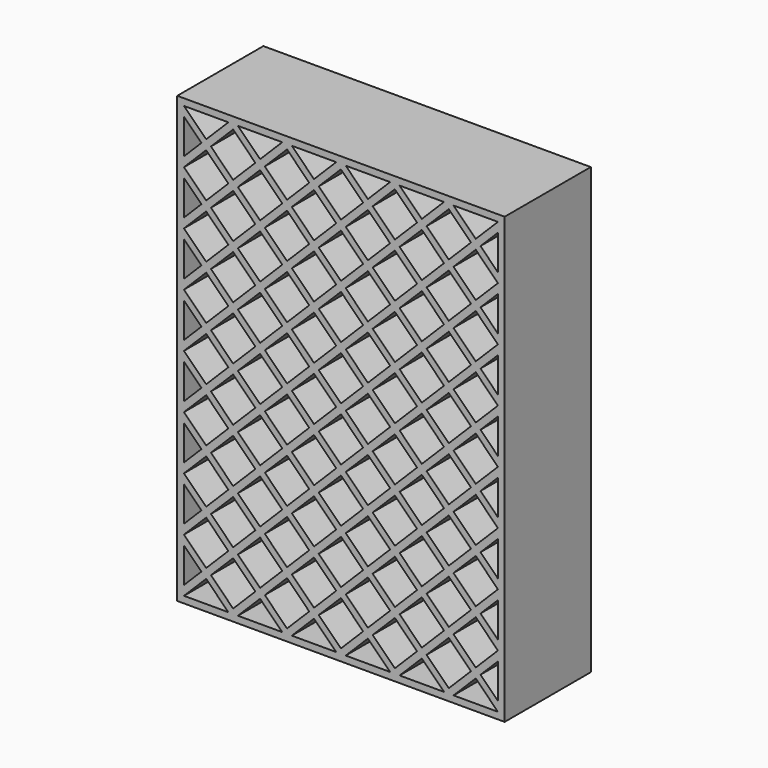
from build123d import *

# Parameters (mm, degrees)
F0_W     = 927.1
F0_H     = 1259.3694764796
F1_DEPTH = 152.4


with BuildPart() as f1:
    # F0 (on Front) → F1 (new body, symmetric)
    with BuildSketch(Plane.XZ):
        with Locations((444.5, 610.6347382398)):
            Rectangle(F0_W, F0_H)
        Polygon((125.6782297091, 0), (0, 0), (0, 26.9407683632), (0, 125.6782297091), (0, 152.6189980723), (0, 152.6643540582), (0, 179.6051224214), (0, 278.3425837673), (0, 305.2833521305), (0, 305.3287081164), (0, 332.2694764796), (0, 431.0069378255), (0, 457.9477061887), (0, 457.9930621745), (0, 484.9338305377), (0, 583.6712918836), (0, 610.6120602469), (0, 610.6574162327), (0, 637.5981845959), (0, 736.3356459418), (0, 763.276414305), (0, 763.3217702909), (0, 790.2625386541), (0, 889), (0, 915.9407683632), (0, 915.9861243491), (0, 942.9268927123), (0, 1041.6643540582), (0, 1068.6051224214), (0, 1068.6504784072), (0, 1095.5912467704), (0, 1194.3287081164), (0, 1221.2694764796), (125.6782297091, 1221.2694764796), (125.700907702, 1221.2921544725), (125.723585695, 1221.2694764796), (152.6189980723, 1221.2694764796), (152.6416760653, 1221.2921544725), (152.6643540582, 1221.2694764796), (278.3425837673, 1221.2694764796), (278.3652617602, 1221.2921544725), (278.3879397531, 1221.2694764796), (305.2833521305, 1221.2694764796), (305.3060301234, 1221.2921544725), (305.3287081164, 1221.2694764796), (431.0069378255, 1221.2694764796), (431.0296158184, 1221.2921544725), (431.0522938113, 1221.2694764796), (457.9477061887, 1221.2694764796), (457.9703841816, 1221.2921544725), (457.9930621745, 1221.2694764796), (583.6712918836, 1221.2694764796), (583.6939698766, 1221.2921544725), (583.7166478695, 1221.2694764796), (610.6120602469, 1221.2694764796), (610.6347382398, 1221.2921544725), (610.6574162327, 1221.2694764796), (736.3356459418, 1221.2694764796), (736.3583239347, 1221.2921544725), (736.3810019277, 1221.2694764796), (763.276414305, 1221.2694764796), (763.299092298, 1221.2921544725), (763.3217702909, 1221.2694764796), (889, 1221.2694764796), (889, 1194.3287081164), (889, 1095.5912467704), (889, 1068.6504784072), (889, 1068.6051224214), (889, 1041.6643540582), (889, 942.9268927123), (889, 915.9861243491), (889, 915.9407683632), (889, 889), (889, 790.2625386541), (889, 763.3217702909), (889, 763.276414305), (889, 736.3356459418), (889, 637.5981845959), (889, 610.6574162327), (889, 610.6120602469), (889, 583.6712918836), (889, 484.9338305377), (889, 457.9930621745), (889, 457.9477061887), (889, 431.0069378255), (889, 332.2694764796), (889, 305.3287081164), (889, 305.2833521305), (889, 278.3425837673), (889, 179.6051224214), (889, 152.6643540582), (889, 152.6189980723), (889, 125.6782297091), (889, 26.9407683632), (889, 0), (763.3217702909, 0), (763.276414305, 0), (736.3810019277, 0), (736.3356459418, 0), (610.6574162327, 0), (610.6120602469, 0), (583.7166478695, 0), (583.6712918836, 0), (457.9930621745, 0), (457.9477061887, 0), (431.0522938113, 0), (431.0069378255, 0), (305.3287081164, 0), (305.2833521305, 0), (278.3879397531, 0), (278.3425837673, 0), (152.6643540582, 0), (152.6189980723, 0), (125.723585695, 0), align=None, mode=Mode.SUBTRACT)
        Polygon((125.700907702, 915.9634463561), (139.1712918836, 902.4930621745), (152.6416760653, 915.9634463561), (139.1712918836, 929.4338305377), align=None)
        Polygon((125.700907702, 1068.6278004143), (139.1712918836, 1055.1574162327), (152.6416760653, 1068.6278004143), (139.1712918836, 1082.0981845959), align=None)
        Polygon((291.8356459418, 1082.0981845959), (305.3060301234, 1068.6278004143), (368.1678229709, 1131.4895932618), (354.6974387893, 1144.9599774434), align=None)
        Polygon((125.700907702, 763.299092298), (139.1712918836, 749.8287081164), (152.6416760653, 763.299092298), (139.1712918836, 776.7694764796), align=None)
        Polygon((291.8356459418, 776.7694764796), (305.3060301234, 763.299092298), (368.1678229709, 826.1608851454), (354.6974387893, 839.631269327), align=None)
        Polygon((291.8356459418, 902.4930621745), (354.6974387893, 839.631269327), (368.1678229709, 853.1016535086), (305.3060301234, 915.9634463561), align=None)
        Polygon((354.6974387893, 992.2956233852), (368.1678229709, 978.8252392036), (381.6382071525, 992.2956233852), (368.1678229709, 1005.7660075668), align=None)
        Polygon((62.8391148546, 853.1016535086), (76.3094990362, 839.631269327), (139.1712918836, 902.4930621745), (125.700907702, 915.9634463561), align=None)
        Polygon((49.368730673, 1144.9599774434), (62.8391148546, 1131.4895932618), (76.3094990362, 1144.9599774434), (62.8391148546, 1158.430361625), align=None)
        Polygon((215.5034689127, 978.8252392036), (278.3652617602, 915.9634463561), (291.8356459418, 929.4338305377), (228.9738530943, 992.2956233852), align=None)
        Polygon((278.3652617602, 1068.6278004143), (291.8356459418, 1055.1574162327), (305.3060301234, 1068.6278004143), (291.8356459418, 1082.0981845959), align=None)
        Polygon((62.8391148546, 826.1608851454), (125.700907702, 763.299092298), (139.1712918836, 776.7694764796), (76.3094990362, 839.631269327), align=None)
        Polygon((49.368730673, 992.2956233852), (62.8391148546, 978.8252392036), (76.3094990362, 992.2956233852), (62.8391148546, 1005.7660075668), align=None)
        Polygon((215.5034689127, 826.1608851454), (278.3652617602, 763.299092298), (291.8356459418, 776.7694764796), (228.9738530943, 839.631269327), align=None)
        Polygon((278.3652617602, 915.9634463561), (291.8356459418, 902.4930621745), (305.3060301234, 915.9634463561), (291.8356459418, 929.4338305377), align=None)
        Polygon((354.6974387893, 1144.9599774434), (368.1678229709, 1131.4895932618), (381.6382071525, 1144.9599774434), (368.1678229709, 1158.430361625), align=None)
        Polygon((139.1712918836, 902.4930621745), (202.0330847311, 839.631269327), (215.5034689127, 853.1016535086), (152.6416760653, 915.9634463561), align=None)
        Polygon((62.8391148546, 978.8252392036), (125.700907702, 915.9634463561), (139.1712918836, 929.4338305377), (76.3094990362, 992.2956233852), align=None)
        Polygon((215.5034689127, 1005.7660075668), (228.9738530943, 992.2956233852), (291.8356459418, 1055.1574162327), (278.3652617602, 1068.6278004143), align=None)
        Polygon((215.5034689127, 853.1016535086), (228.9738530943, 839.631269327), (291.8356459418, 902.4930621745), (278.3652617602, 915.9634463561), align=None)
        Polygon((278.3652617602, 763.299092298), (291.8356459418, 749.8287081164), (305.3060301234, 763.299092298), (291.8356459418, 776.7694764796), align=None)
        Polygon((291.8356459418, 929.4338305377), (305.3060301234, 915.9634463561), (368.1678229709, 978.8252392036), (354.6974387893, 992.2956233852), align=None)
        Polygon((49.368730673, 839.631269327), (62.8391148546, 826.1608851454), (76.3094990362, 839.631269327), (62.8391148546, 853.1016535086), align=None)
        Polygon((62.8391148546, 1005.7660075668), (76.3094990362, 992.2956233852), (139.1712918836, 1055.1574162327), (125.700907702, 1068.6278004143), align=None)
        Polygon((62.8391148546, 1131.4895932618), (125.700907702, 1068.6278004143), (139.1712918836, 1082.0981845959), (76.3094990362, 1144.9599774434), align=None)
        Polygon((202.0330847311, 992.2956233852), (215.5034689127, 978.8252392036), (228.9738530943, 992.2956233852), (215.5034689127, 1005.7660075668), align=None)
        Polygon((202.0330847311, 839.631269327), (215.5034689127, 826.1608851454), (228.9738530943, 839.631269327), (215.5034689127, 853.1016535086), align=None)
        Polygon((202.0330847311, 1144.9599774434), (215.5034689127, 1131.4895932618), (228.9738530943, 1144.9599774434), (215.5034689127, 1158.430361625), align=None)
        Polygon((139.1712918836, 929.4338305377), (152.6416760653, 915.9634463561), (215.5034689127, 978.8252392036), (202.0330847311, 992.2956233852), align=None)
        Polygon((139.1712918836, 1055.1574162327), (202.0330847311, 992.2956233852), (215.5034689127, 1005.7660075668), (152.6416760653, 1068.6278004143), align=None)
        Polygon((139.1712918836, 1082.0981845959), (152.6416760653, 1068.6278004143), (215.5034689127, 1131.4895932618), (202.0330847311, 1144.9599774434), align=None)
        Polygon((354.6974387893, 839.631269327), (368.1678229709, 826.1608851454), (381.6382071525, 839.631269327), (368.1678229709, 853.1016535086), align=None)
        Polygon((215.5034689127, 1131.4895932618), (278.3652617602, 1068.6278004143), (291.8356459418, 1082.0981845959), (228.9738530943, 1144.9599774434), align=None)
        Polygon((291.8356459418, 1055.1574162327), (354.6974387893, 992.2956233852), (368.1678229709, 1005.7660075668), (305.3060301234, 1068.6278004143), align=None)
        Polygon((139.1712918836, 776.7694764796), (152.6416760653, 763.299092298), (215.5034689127, 826.1608851454), (202.0330847311, 839.631269327), align=None)
        Polygon((139.1712918836, 444.5), (202.0330847311, 381.6382071525), (215.5034689127, 395.1085913341), (152.6416760653, 457.9703841816), align=None)
        Polygon((431.0296158184, 152.6416760653), (368.1678229709, 89.7798832178), (381.6382071525, 76.3094990362), (444.5, 139.1712918836), align=None)
        Polygon((749.8287081164, 1055.1574162327), (812.6905009638, 992.2956233852), (826.1608851454, 1005.7660075668), (763.299092298, 1068.6278004143), align=None)
        Polygon((597.1643540582, 929.4338305377), (610.6347382398, 915.9634463561), (673.4965310873, 978.8252392036), (660.0261469057, 992.2956233852), align=None)
        Polygon((444.5, 902.4930621745), (507.3617928475, 839.631269327), (520.8321770291, 853.1016535086), (457.9703841816, 915.9634463561), align=None)
        Polygon((610.6347382398, 152.6416760653), (597.1643540582, 139.1712918836), (660.0261469057, 76.3094990362), (673.4965310873, 89.7798832178), align=None)
        Polygon((291.8356459418, 13.4477061887), (305.2833521305, 0), (305.3287081164, 0), (368.1678229709, 62.8391148546), (354.6974387893, 76.3094990362), align=None)
        Polygon((368.1678229709, 395.1085913341), (381.6382071525, 381.6382071525), (444.5, 444.5), (431.0296158184, 457.9703841816), align=None)
        Polygon((583.6939698766, 305.3060301234), (520.8321770291, 242.4442372759), (534.3025612107, 228.9738530943), (597.1643540582, 291.8356459418), align=None)
        Polygon((673.4965310873, 700.4372994505), (686.9669152689, 686.9669152689), (749.8287081164, 749.8287081164), (736.3583239347, 763.299092298), align=None)
        Polygon((444.5, 597.1643540582), (507.3617928475, 534.3025612107), (520.8321770291, 547.7729453923), (457.9703841816, 610.6347382398), align=None)
        Polygon((291.8356459418, 471.4407683632), (305.3060301234, 457.9703841816), (368.1678229709, 520.8321770291), (354.6974387893, 534.3025612107), align=None)
        Polygon((0, 152.6189980723), (0, 125.6782297091), (49.368730673, 76.3094990362), (62.8391148546, 89.7798832178), align=None)
        Polygon((889, 152.6189980723), (826.1608851454, 89.7798832178), (839.631269327, 76.3094990362), (889, 125.6782297091), align=None)
        Polygon((749.8287081164, 13.4477061887), (763.276414305, 0), (763.3217702909, 0), (826.1608851454, 62.8391148546), (812.6905009638, 76.3094990362), align=None)
        Polygon((763.299092298, 152.6416760653), (749.8287081164, 139.1712918836), (812.6905009638, 76.3094990362), (826.1608851454, 89.7798832178), align=None)
        Polygon((431.0296158184, 763.299092298), (444.5, 749.8287081164), (457.9703841816, 763.299092298), (444.5, 776.7694764796), align=None)
        Polygon((62.8391148546, 89.7798832178), (76.3094990362, 76.3094990362), (139.1712918836, 139.1712918836), (125.700907702, 152.6416760653), align=None)
        Polygon((673.4965310873, 242.4442372759), (660.0261469057, 228.9738530943), (673.4965310873, 215.5034689127), (686.9669152689, 228.9738530943), align=None)
        Polygon((812.6905009638, 228.9738530943), (749.8287081164, 166.1120602469), (763.299092298, 152.6416760653), (826.1608851454, 215.5034689127), align=None)
        Polygon((0, 790.2625386541), (0, 763.3217702909), (62.8391148546, 826.1608851454), (49.368730673, 839.631269327), align=None)
        Polygon((368.1678229709, 1158.430361625), (381.6382071525, 1144.9599774434), (444.5, 1207.8217702909), (431.0522938113, 1221.2694764796), (431.0069378255, 1221.2694764796), align=None)
        Polygon((215.5034689127, 89.7798832178), (202.0330847311, 76.3094990362), (215.5034689127, 62.8391148546), (228.9738530943, 76.3094990362), align=None)
        Polygon((354.6974387893, 686.9669152689), (368.1678229709, 673.4965310873), (381.6382071525, 686.9669152689), (368.1678229709, 700.4372994505), align=None)
        Polygon((597.1643540582, 471.4407683632), (583.6939698766, 457.9703841816), (597.1643540582, 444.5), (610.6347382398, 457.9703841816), align=None)
        Polygon((49.368730673, 228.9738530943), (62.8391148546, 215.5034689127), (76.3094990362, 228.9738530943), (62.8391148546, 242.4442372759), align=None)
        Polygon((139.1712918836, 597.1643540582), (202.0330847311, 534.3025612107), (215.5034689127, 547.7729453923), (152.6416760653, 610.6347382398), align=None)
        Polygon((660.0261469057, 1144.9599774434), (673.4965310873, 1131.4895932618), (686.9669152689, 1144.9599774434), (673.4965310873, 1158.430361625), align=None)
        Polygon((62.8391148546, 700.4372994505), (76.3094990362, 686.9669152689), (139.1712918836, 749.8287081164), (125.700907702, 763.299092298), align=None)
        Polygon((749.8287081164, 902.4930621745), (812.6905009638, 839.631269327), (826.1608851454, 853.1016535086), (763.299092298, 915.9634463561), align=None)
        Polygon((597.1643540582, 776.7694764796), (610.6347382398, 763.299092298), (673.4965310873, 826.1608851454), (660.0261469057, 839.631269327), align=None)
        Polygon((444.5, 749.8287081164), (507.3617928475, 686.9669152689), (520.8321770291, 700.4372994505), (457.9703841816, 763.299092298), align=None)
        Polygon((291.8356459418, 624.1051224214), (305.3060301234, 610.6347382398), (368.1678229709, 673.4965310873), (354.6974387893, 686.9669152689), align=None)
        Polygon((610.6347382398, 457.9703841816), (597.1643540582, 444.5), (660.0261469057, 381.6382071525), (673.4965310873, 395.1085913341), align=None)
        Polygon((826.1608851454, 700.4372994505), (812.6905009638, 686.9669152689), (826.1608851454, 673.4965310873), (839.631269327, 686.9669152689), align=None)
        Polygon((812.6905009638, 534.3025612107), (749.8287081164, 471.4407683632), (763.299092298, 457.9703841816), (826.1608851454, 520.8321770291), align=None)
        Polygon((812.6905009638, 1144.9599774434), (826.1608851454, 1131.4895932618), (839.631269327, 1144.9599774434), (826.1608851454, 1158.430361625), align=None)
        Polygon((520.8321770291, 1005.7660075668), (534.3025612107, 992.2956233852), (597.1643540582, 1055.1574162327), (583.6939698766, 1068.6278004143), align=None)
        Polygon((0, 610.6120602469), (0, 583.6712918836), (49.368730673, 534.3025612107), (62.8391148546, 547.7729453923), align=None)
        Polygon((520.8321770291, 1131.4895932618), (583.6939698766, 1068.6278004143), (597.1643540582, 1082.0981845959), (534.3025612107, 1144.9599774434), align=None)
        Polygon((507.3617928475, 686.9669152689), (520.8321770291, 673.4965310873), (534.3025612107, 686.9669152689), (520.8321770291, 700.4372994505), align=None)
        Polygon((202.0330847311, 534.3025612107), (215.5034689127, 520.8321770291), (228.9738530943, 534.3025612107), (215.5034689127, 547.7729453923), align=None)
        Polygon((673.4965310873, 1158.430361625), (686.9669152689, 1144.9599774434), (749.8287081164, 1207.8217702909), (736.3810019277, 1221.2694764796), (736.3356459418, 1221.2694764796), align=None)
        Polygon((839.631269327, 534.3025612107), (826.1608851454, 520.8321770291), (889, 457.9930621745), (889, 484.9338305377), align=None)
        Polygon((812.6905009638, 839.631269327), (826.1608851454, 826.1608851454), (839.631269327, 839.631269327), (826.1608851454, 853.1016535086), align=None)
        Polygon((583.6939698766, 915.9634463561), (597.1643540582, 902.4930621745), (610.6347382398, 915.9634463561), (597.1643540582, 929.4338305377), align=None)
        Polygon((381.6382071525, 381.6382071525), (368.1678229709, 368.1678229709), (431.0296158184, 305.3060301234), (444.5, 318.776414305), align=None)
        Polygon((0, 915.9407683632), (0, 889), (49.368730673, 839.631269327), (62.8391148546, 853.1016535086), align=None)
        Polygon((686.9669152689, 686.9669152689), (673.4965310873, 673.4965310873), (736.3583239347, 610.6347382398), (749.8287081164, 624.1051224214), align=None)
        Polygon((278.3652617602, 457.9703841816), (291.8356459418, 444.5), (305.3060301234, 457.9703841816), (291.8356459418, 471.4407683632), align=None)
        Polygon((215.5034689127, 62.8391148546), (278.3425837673, 0), (278.3879397531, 0), (291.8356459418, 13.4477061887), (228.9738530943, 76.3094990362), align=None)
        Polygon((0, 26.9407683632), (0, 0), (62.8391148546, 62.8391148546), (49.368730673, 76.3094990362), align=None)
        Polygon((889, 763.276414305), (826.1608851454, 700.4372994505), (839.631269327, 686.9669152689), (889, 736.3356459418), align=None)
        Polygon((826.1608851454, 62.8391148546), (889, 0), (889, 26.9407683632), (839.631269327, 76.3094990362), align=None)
        Polygon((49.368730673, 76.3094990362), (62.8391148546, 62.8391148546), (76.3094990362, 76.3094990362), (62.8391148546, 89.7798832178), align=None)
        Polygon((812.6905009638, 686.9669152689), (749.8287081164, 624.1051224214), (763.299092298, 610.6347382398), (826.1608851454, 673.4965310873), align=None)
        Polygon((534.3025612107, 228.9738530943), (520.8321770291, 215.5034689127), (583.6939698766, 152.6416760653), (597.1643540582, 166.1120602469), align=None)
        Polygon((368.1678229709, 89.7798832178), (354.6974387893, 76.3094990362), (368.1678229709, 62.8391148546), (381.6382071525, 76.3094990362), align=None)
        Polygon((215.5034689127, 242.4442372759), (228.9738530943, 228.9738530943), (291.8356459418, 291.8356459418), (278.3652617602, 305.3060301234), align=None)
        Polygon((520.8321770291, 547.7729453923), (534.3025612107, 534.3025612107), (597.1643540582, 597.1643540582), (583.6939698766, 610.6347382398), align=None)
        Polygon((139.1712918836, 291.8356459418), (202.0330847311, 228.9738530943), (215.5034689127, 242.4442372759), (152.6416760653, 305.3060301234), align=None)
        Polygon((0, 763.276414305), (0, 736.3356459418), (49.368730673, 686.9669152689), (62.8391148546, 700.4372994505), align=None)
        Polygon((507.3617928475, 992.2956233852), (520.8321770291, 978.8252392036), (534.3025612107, 992.2956233852), (520.8321770291, 1005.7660075668), align=None)
        Polygon((520.8321770291, 242.4442372759), (507.3617928475, 228.9738530943), (520.8321770291, 215.5034689127), (534.3025612107, 228.9738530943), align=None)
        Polygon((686.9669152689, 381.6382071525), (673.4965310873, 368.1678229709), (736.3583239347, 305.3060301234), (749.8287081164, 318.776414305), align=None)
        Polygon((520.8321770291, 62.8391148546), (583.6712918836, 0), (583.7166478695, 0), (597.1643540582, 13.4477061887), (534.3025612107, 76.3094990362), align=None)
        Polygon((354.6974387893, 228.9738530943), (291.8356459418, 166.1120602469), (305.3060301234, 152.6416760653), (368.1678229709, 215.5034689127), align=None)
        Polygon((583.6939698766, 763.299092298), (597.1643540582, 749.8287081164), (610.6347382398, 763.299092298), (597.1643540582, 776.7694764796), align=None)
        Polygon((278.3652617602, 610.6347382398), (291.8356459418, 597.1643540582), (305.3060301234, 610.6347382398), (291.8356459418, 624.1051224214), align=None)
        Polygon((839.631269327, 686.9669152689), (826.1608851454, 673.4965310873), (889, 610.6574162327), (889, 637.5981845959), align=None)
        Polygon((228.9738530943, 228.9738530943), (215.5034689127, 215.5034689127), (278.3652617602, 152.6416760653), (291.8356459418, 166.1120602469), align=None)
        Polygon((534.3025612107, 534.3025612107), (520.8321770291, 520.8321770291), (583.6939698766, 457.9703841816), (597.1643540582, 471.4407683632), align=None)
        Polygon((444.5, 166.1120602469), (431.0296158184, 152.6416760653), (444.5, 139.1712918836), (457.9703841816, 152.6416760653), align=None)
        Polygon((291.8356459418, 597.1643540582), (354.6974387893, 534.3025612107), (368.1678229709, 547.7729453923), (305.3060301234, 610.6347382398), align=None)
        Polygon((139.1712918836, 471.4407683632), (152.6416760653, 457.9703841816), (215.5034689127, 520.8321770291), (202.0330847311, 534.3025612107), align=None)
        Polygon((444.5, 471.4407683632), (457.9703841816, 457.9703841816), (520.8321770291, 520.8321770291), (507.3617928475, 534.3025612107), align=None)
        Polygon((749.8287081164, 1082.0981845959), (763.299092298, 1068.6278004143), (826.1608851454, 1131.4895932618), (812.6905009638, 1144.9599774434), align=None)
        Polygon((597.1643540582, 1055.1574162327), (660.0261469057, 992.2956233852), (673.4965310873, 1005.7660075668), (610.6347382398, 1068.6278004143), align=None)
        Polygon((749.8287081164, 776.7694764796), (763.299092298, 763.299092298), (826.1608851454, 826.1608851454), (812.6905009638, 839.631269327), align=None)
        Polygon((597.1643540582, 749.8287081164), (660.0261469057, 686.9669152689), (673.4965310873, 700.4372994505), (610.6347382398, 763.299092298), align=None)
        Polygon((597.1643540582, 166.1120602469), (583.6939698766, 152.6416760653), (597.1643540582, 139.1712918836), (610.6347382398, 152.6416760653), align=None)
        Polygon((444.5, 624.1051224214), (457.9703841816, 610.6347382398), (520.8321770291, 673.4965310873), (507.3617928475, 686.9669152689), align=None)
        Polygon((610.6347382398, 305.3060301234), (597.1643540582, 291.8356459418), (660.0261469057, 228.9738530943), (673.4965310873, 242.4442372759), align=None)
        Polygon((0, 457.9477061887), (0, 431.0069378255), (49.368730673, 381.6382071525), (62.8391148546, 395.1085913341), align=None)
        Polygon((368.1678229709, 62.8391148546), (431.0069378255, 0), (431.0522938113, 0), (444.5, 13.4477061887), (381.6382071525, 76.3094990362), align=None)
        Polygon((889, 457.9477061887), (826.1608851454, 395.1085913341), (839.631269327, 381.6382071525), (889, 431.0069378255), align=None)
        Polygon((139.1712918836, 166.1120602469), (152.6416760653, 152.6416760653), (215.5034689127, 215.5034689127), (202.0330847311, 228.9738530943), align=None)
        Polygon((749.8287081164, 166.1120602469), (736.3583239347, 152.6416760653), (749.8287081164, 139.1712918836), (763.299092298, 152.6416760653), align=None)
        Polygon((520.8321770291, 1158.430361625), (534.3025612107, 1144.9599774434), (597.1643540582, 1207.8217702909), (583.7166478695, 1221.2694764796), (583.6712918836, 1221.2694764796), align=None)
        Polygon((534.3025612107, 381.6382071525), (520.8321770291, 368.1678229709), (583.6939698766, 305.3060301234), (597.1643540582, 318.776414305), align=None)
        Polygon((736.3583239347, 457.9703841816), (673.4965310873, 395.1085913341), (686.9669152689, 381.6382071525), (749.8287081164, 444.5), align=None)
        Polygon((520.8321770291, 395.1085913341), (507.3617928475, 381.6382071525), (520.8321770291, 368.1678229709), (534.3025612107, 381.6382071525), align=None)
        Polygon((215.5034689127, 700.4372994505), (228.9738530943, 686.9669152689), (291.8356459418, 749.8287081164), (278.3652617602, 763.299092298), align=None)
        Polygon((826.1608851454, 395.1085913341), (812.6905009638, 381.6382071525), (826.1608851454, 368.1678229709), (839.631269327, 381.6382071525), align=None)
        Polygon((62.8391148546, 1158.430361625), (76.3094990362, 1144.9599774434), (139.1712918836, 1207.8217702909), (125.723585695, 1221.2694764796), (125.6782297091, 1221.2694764796), align=None)
        Polygon((812.6905009638, 992.2956233852), (826.1608851454, 978.8252392036), (839.631269327, 992.2956233852), (826.1608851454, 1005.7660075668), align=None)
        Polygon((139.1712918836, 13.4477061887), (152.6189980723, 0), (152.6643540582, 0), (215.5034689127, 62.8391148546), (202.0330847311, 76.3094990362), align=None)
        Polygon((763.299092298, 610.6347382398), (749.8287081164, 597.1643540582), (812.6905009638, 534.3025612107), (826.1608851454, 547.7729453923), align=None)
        Polygon((507.3617928475, 839.631269327), (520.8321770291, 826.1608851454), (534.3025612107, 839.631269327), (520.8321770291, 853.1016535086), align=None)
        Polygon((749.8287081164, 624.1051224214), (736.3583239347, 610.6347382398), (749.8287081164, 597.1643540582), (763.299092298, 610.6347382398), align=None)
        Polygon((660.0261469057, 839.631269327), (673.4965310873, 826.1608851454), (686.9669152689, 839.631269327), (673.4965310873, 853.1016535086), align=None)
        Polygon((660.0261469057, 381.6382071525), (597.1643540582, 318.776414305), (610.6347382398, 305.3060301234), (673.4965310873, 368.1678229709), align=None)
        Polygon((0, 637.5981845959), (0, 610.6574162327), (62.8391148546, 673.4965310873), (49.368730673, 686.9669152689), align=None)
        Polygon((444.5, 1055.1574162327), (507.3617928475, 992.2956233852), (520.8321770291, 1005.7660075668), (457.9703841816, 1068.6278004143), align=None)
        Polygon((507.3617928475, 228.9738530943), (444.5, 166.1120602469), (457.9703841816, 152.6416760653), (520.8321770291, 215.5034689127), align=None)
        Polygon((444.5, 929.4338305377), (457.9703841816, 915.9634463561), (520.8321770291, 978.8252392036), (507.3617928475, 992.2956233852), align=None)
        Polygon((686.9669152689, 228.9738530943), (673.4965310873, 215.5034689127), (736.3583239347, 152.6416760653), (749.8287081164, 166.1120602469), align=None)
        Polygon((444.5, 13.4477061887), (457.9477061887, 0), (457.9930621745, 0), (520.8321770291, 62.8391148546), (507.3617928475, 76.3094990362), align=None)
        Polygon((291.8356459418, 166.1120602469), (278.3652617602, 152.6416760653), (291.8356459418, 139.1712918836), (305.3060301234, 152.6416760653), align=None)
        Polygon((305.3060301234, 152.6416760653), (291.8356459418, 139.1712918836), (354.6974387893, 76.3094990362), (368.1678229709, 89.7798832178), align=None)
        Polygon((597.1643540582, 1082.0981845959), (610.6347382398, 1068.6278004143), (673.4965310873, 1131.4895932618), (660.0261469057, 1144.9599774434), align=None)
        Polygon((49.368730673, 686.9669152689), (62.8391148546, 673.4965310873), (76.3094990362, 686.9669152689), (62.8391148546, 700.4372994505), align=None)
        Polygon((889, 610.6120602469), (826.1608851454, 547.7729453923), (839.631269327, 534.3025612107), (889, 583.6712918836), align=None)
        Polygon((202.0330847311, 228.9738530943), (215.5034689127, 215.5034689127), (228.9738530943, 228.9738530943), (215.5034689127, 242.4442372759), align=None)
        Polygon((507.3617928475, 534.3025612107), (520.8321770291, 520.8321770291), (534.3025612107, 534.3025612107), (520.8321770291, 547.7729453923), align=None)
        Polygon((62.8391148546, 215.5034689127), (125.700907702, 152.6416760653), (139.1712918836, 166.1120602469), (76.3094990362, 228.9738530943), align=None)
        Polygon((507.3617928475, 1144.9599774434), (520.8321770291, 1131.4895932618), (534.3025612107, 1144.9599774434), (520.8321770291, 1158.430361625), align=None)
        Polygon((278.3652617602, 152.6416760653), (215.5034689127, 89.7798832178), (228.9738530943, 76.3094990362), (291.8356459418, 139.1712918836), align=None)
        Polygon((125.700907702, 457.9703841816), (139.1712918836, 444.5), (152.6416760653, 457.9703841816), (139.1712918836, 471.4407683632), align=None)
        Polygon((673.4965310873, 1131.4895932618), (736.3583239347, 1068.6278004143), (749.8287081164, 1082.0981845959), (686.9669152689, 1144.9599774434), align=None)
        Polygon((457.9703841816, 457.9703841816), (444.5, 444.5), (507.3617928475, 381.6382071525), (520.8321770291, 395.1085913341), align=None)
        Polygon((520.8321770291, 89.7798832178), (507.3617928475, 76.3094990362), (520.8321770291, 62.8391148546), (534.3025612107, 76.3094990362), align=None)
        Polygon((62.8391148546, 520.8321770291), (125.700907702, 457.9703841816), (139.1712918836, 471.4407683632), (76.3094990362, 534.3025612107), align=None)
        Polygon((763.299092298, 763.299092298), (749.8287081164, 749.8287081164), (812.6905009638, 686.9669152689), (826.1608851454, 700.4372994505), align=None)
        Polygon((202.0330847311, 381.6382071525), (215.5034689127, 368.1678229709), (228.9738530943, 381.6382071525), (215.5034689127, 395.1085913341), align=None)
        Polygon((0, 1095.5912467704), (0, 1068.6504784072), (62.8391148546, 1131.4895932618), (49.368730673, 1144.9599774434), align=None)
        Polygon((839.631269327, 1144.9599774434), (826.1608851454, 1131.4895932618), (889, 1068.6504784072), (889, 1095.5912467704), align=None)
        Polygon((583.6939698766, 152.6416760653), (520.8321770291, 89.7798832178), (534.3025612107, 76.3094990362), (597.1643540582, 139.1712918836), align=None)
        Polygon((597.1643540582, 1207.8217702909), (660.0261469057, 1144.9599774434), (673.4965310873, 1158.430361625), (610.6574162327, 1221.2694764796), (610.6120602469, 1221.2694764796), align=None)
        Polygon((507.3617928475, 381.6382071525), (444.5, 318.776414305), (457.9703841816, 305.3060301234), (520.8321770291, 368.1678229709), align=None)
        Polygon((673.4965310873, 395.1085913341), (660.0261469057, 381.6382071525), (673.4965310873, 368.1678229709), (686.9669152689, 381.6382071525), align=None)
        Polygon((202.0330847311, 686.9669152689), (215.5034689127, 673.4965310873), (228.9738530943, 686.9669152689), (215.5034689127, 700.4372994505), align=None)
        Polygon((368.1678229709, 1131.4895932618), (431.0296158184, 1068.6278004143), (444.5, 1082.0981845959), (381.6382071525, 1144.9599774434), align=None)
        Polygon((749.8287081164, 929.4338305377), (763.299092298, 915.9634463561), (826.1608851454, 978.8252392036), (812.6905009638, 992.2956233852), align=None)
        Polygon((444.5, 776.7694764796), (457.9703841816, 763.299092298), (520.8321770291, 826.1608851454), (507.3617928475, 839.631269327), align=None)
        Polygon((597.1643540582, 902.4930621745), (660.0261469057, 839.631269327), (673.4965310873, 853.1016535086), (610.6347382398, 915.9634463561), align=None)
        Polygon((291.8356459418, 749.8287081164), (354.6974387893, 686.9669152689), (368.1678229709, 700.4372994505), (305.3060301234, 763.299092298), align=None)
        Polygon((291.8356459418, 318.776414305), (305.3060301234, 305.3060301234), (368.1678229709, 368.1678229709), (354.6974387893, 381.6382071525), align=None)
        Polygon((597.1643540582, 624.1051224214), (610.6347382398, 610.6347382398), (673.4965310873, 673.4965310873), (660.0261469057, 686.9669152689), align=None)
        Polygon((291.8356459418, 444.5), (354.6974387893, 381.6382071525), (368.1678229709, 395.1085913341), (305.3060301234, 457.9703841816), align=None)
        Polygon((62.8391148546, 673.4965310873), (125.700907702, 610.6347382398), (139.1712918836, 624.1051224214), (76.3094990362, 686.9669152689), align=None)
        Polygon((139.1712918836, 318.776414305), (152.6416760653, 305.3060301234), (215.5034689127, 368.1678229709), (202.0330847311, 381.6382071525), align=None)
        Polygon((0, 1068.6051224214), (0, 1041.6643540582), (49.368730673, 992.2956233852), (62.8391148546, 1005.7660075668), align=None)
        Polygon((826.1608851454, 1005.7660075668), (839.631269327, 992.2956233852), (889, 1041.6643540582), (889, 1068.6051224214), align=None)
        Polygon((583.6939698766, 1068.6278004143), (597.1643540582, 1055.1574162327), (610.6347382398, 1068.6278004143), (597.1643540582, 1082.0981845959), align=None)
        Polygon((431.0296158184, 610.6347382398), (444.5, 597.1643540582), (457.9703841816, 610.6347382398), (444.5, 624.1051224214), align=None)
        Polygon((673.4965310873, 826.1608851454), (736.3583239347, 763.299092298), (749.8287081164, 776.7694764796), (686.9669152689, 839.631269327), align=None)
        Polygon((520.8321770291, 700.4372994505), (534.3025612107, 686.9669152689), (597.1643540582, 749.8287081164), (583.6939698766, 763.299092298), align=None)
        Polygon((0, 332.2694764796), (0, 305.3287081164), (62.8391148546, 368.1678229709), (49.368730673, 381.6382071525), align=None)
        Polygon((763.299092298, 305.3060301234), (749.8287081164, 291.8356459418), (812.6905009638, 228.9738530943), (826.1608851454, 242.4442372759), align=None)
        Polygon((673.4965310873, 978.8252392036), (736.3583239347, 915.9634463561), (749.8287081164, 929.4338305377), (686.9669152689, 992.2956233852), align=None)
        Polygon((368.1678229709, 826.1608851454), (431.0296158184, 763.299092298), (444.5, 776.7694764796), (381.6382071525, 839.631269327), align=None)
        Polygon((520.8321770291, 853.1016535086), (534.3025612107, 839.631269327), (597.1643540582, 902.4930621745), (583.6939698766, 915.9634463561), align=None)
        Polygon((660.0261469057, 686.9669152689), (673.4965310873, 673.4965310873), (686.9669152689, 686.9669152689), (673.4965310873, 700.4372994505), align=None)
        Polygon((368.1678229709, 520.8321770291), (431.0296158184, 457.9703841816), (444.5, 471.4407683632), (381.6382071525, 534.3025612107), align=None)
        Polygon((215.5034689127, 395.1085913341), (228.9738530943, 381.6382071525), (291.8356459418, 444.5), (278.3652617602, 457.9703841816), align=None)
        Polygon((62.8391148546, 368.1678229709), (125.700907702, 305.3060301234), (139.1712918836, 318.776414305), (76.3094990362, 381.6382071525), align=None)
        Polygon((62.8391148546, 547.7729453923), (76.3094990362, 534.3025612107), (139.1712918836, 597.1643540582), (125.700907702, 610.6347382398), align=None)
        Polygon((0, 1221.2694764796), (0, 1194.3287081164), (49.368730673, 1144.9599774434), (62.8391148546, 1158.430361625), align=None)
        Polygon((826.1608851454, 1158.430361625), (839.631269327, 1144.9599774434), (889, 1194.3287081164), (889, 1221.2694764796), align=None)
        Polygon((354.6974387893, 381.6382071525), (368.1678229709, 368.1678229709), (381.6382071525, 381.6382071525), (368.1678229709, 395.1085913341), align=None)
        Polygon((736.3583239347, 152.6416760653), (673.4965310873, 89.7798832178), (686.9669152689, 76.3094990362), (749.8287081164, 139.1712918836), align=None)
        Polygon((444.5, 1207.8217702909), (507.3617928475, 1144.9599774434), (520.8321770291, 1158.430361625), (457.9930621745, 1221.2694764796), (457.9477061887, 1221.2694764796), align=None)
        Polygon((583.6939698766, 457.9703841816), (520.8321770291, 395.1085913341), (534.3025612107, 381.6382071525), (597.1643540582, 444.5), align=None)
        Polygon((749.8287081164, 471.4407683632), (736.3583239347, 457.9703841816), (749.8287081164, 444.5), (763.299092298, 457.9703841816), align=None)
        Polygon((660.0261469057, 228.9738530943), (597.1643540582, 166.1120602469), (610.6347382398, 152.6416760653), (673.4965310873, 215.5034689127), align=None)
        Polygon((597.1643540582, 13.4477061887), (610.6120602469, 0), (610.6574162327, 0), (673.4965310873, 62.8391148546), (660.0261469057, 76.3094990362), align=None)
        Polygon((839.631269327, 381.6382071525), (826.1608851454, 368.1678229709), (889, 305.3287081164), (889, 332.2694764796), align=None)
        Polygon((152.6416760653, 152.6416760653), (139.1712918836, 139.1712918836), (202.0330847311, 76.3094990362), (215.5034689127, 89.7798832178), align=None)
        Polygon((368.1678229709, 673.4965310873), (431.0296158184, 610.6347382398), (444.5, 624.1051224214), (381.6382071525, 686.9669152689), align=None)
        Polygon((215.5034689127, 547.7729453923), (228.9738530943, 534.3025612107), (291.8356459418, 597.1643540582), (278.3652617602, 610.6347382398), align=None)
        Polygon((749.8287081164, 1207.8217702909), (812.6905009638, 1144.9599774434), (826.1608851454, 1158.430361625), (763.3217702909, 1221.2694764796), (763.276414305, 1221.2694764796), align=None)
        Polygon((812.6905009638, 381.6382071525), (749.8287081164, 318.776414305), (763.299092298, 305.3060301234), (826.1608851454, 368.1678229709), align=None)
        Polygon((62.8391148546, 62.8391148546), (125.6782297091, 0), (125.723585695, 0), (139.1712918836, 13.4477061887), (76.3094990362, 76.3094990362), align=None)
        Polygon((139.1712918836, 1207.8217702909), (202.0330847311, 1144.9599774434), (215.5034689127, 1158.430361625), (152.6643540582, 1221.2694764796), (152.6189980723, 1221.2694764796), align=None)
        Polygon((736.3583239347, 610.6347382398), (673.4965310873, 547.7729453923), (686.9669152689, 534.3025612107), (749.8287081164, 597.1643540582), align=None)
        Polygon((457.9703841816, 152.6416760653), (444.5, 139.1712918836), (507.3617928475, 76.3094990362), (520.8321770291, 89.7798832178), align=None)
        Polygon((431.0296158184, 915.9634463561), (444.5, 902.4930621745), (457.9703841816, 915.9634463561), (444.5, 929.4338305377), align=None)
        Polygon((444.5, 1082.0981845959), (457.9703841816, 1068.6278004143), (520.8321770291, 1131.4895932618), (507.3617928475, 1144.9599774434), align=None)
        Polygon((215.5034689127, 520.8321770291), (278.3652617602, 457.9703841816), (291.8356459418, 471.4407683632), (228.9738530943, 534.3025612107), align=None)
        Polygon((62.8391148546, 395.1085913341), (76.3094990362, 381.6382071525), (139.1712918836, 444.5), (125.700907702, 457.9703841816), align=None)
        Polygon((673.4965310873, 1005.7660075668), (686.9669152689, 992.2956233852), (749.8287081164, 1055.1574162327), (736.3583239347, 1068.6278004143), align=None)
        Polygon((520.8321770291, 978.8252392036), (583.6939698766, 915.9634463561), (597.1643540582, 929.4338305377), (534.3025612107, 992.2956233852), align=None)
        Polygon((431.0296158184, 457.9703841816), (444.5, 444.5), (457.9703841816, 457.9703841816), (444.5, 471.4407683632), align=None)
        Polygon((736.3583239347, 763.299092298), (749.8287081164, 749.8287081164), (763.299092298, 763.299092298), (749.8287081164, 776.7694764796), align=None)
        Polygon((520.8321770291, 673.4965310873), (583.6939698766, 610.6347382398), (597.1643540582, 624.1051224214), (534.3025612107, 686.9669152689), align=None)
        Polygon((368.1678229709, 547.7729453923), (381.6382071525, 534.3025612107), (444.5, 597.1643540582), (431.0296158184, 610.6347382398), align=None)
        Polygon((0, 305.2833521305), (0, 278.3425837673), (49.368730673, 228.9738530943), (62.8391148546, 242.4442372759), align=None)
        Polygon((889, 305.2833521305), (826.1608851454, 242.4442372759), (839.631269327, 228.9738530943), (889, 278.3425837673), align=None)
        Polygon((125.700907702, 152.6416760653), (139.1712918836, 139.1712918836), (152.6416760653, 152.6416760653), (139.1712918836, 166.1120602469), align=None)
        Polygon((749.8287081164, 318.776414305), (736.3583239347, 305.3060301234), (749.8287081164, 291.8356459418), (763.299092298, 305.3060301234), align=None)
        Polygon((673.4965310873, 89.7798832178), (660.0261469057, 76.3094990362), (673.4965310873, 62.8391148546), (686.9669152689, 76.3094990362), align=None)
        Polygon((215.5034689127, 1158.430361625), (228.9738530943, 1144.9599774434), (291.8356459418, 1207.8217702909), (278.3879397531, 1221.2694764796), (278.3425837673, 1221.2694764796), align=None)
        Polygon((583.6939698766, 610.6347382398), (597.1643540582, 597.1643540582), (610.6347382398, 610.6347382398), (597.1643540582, 624.1051224214), align=None)
        Polygon((686.9669152689, 534.3025612107), (673.4965310873, 520.8321770291), (736.3583239347, 457.9703841816), (749.8287081164, 471.4407683632), align=None)
        Polygon((368.1678229709, 853.1016535086), (381.6382071525, 839.631269327), (444.5, 902.4930621745), (431.0296158184, 915.9634463561), align=None)
        Polygon((368.1678229709, 978.8252392036), (431.0296158184, 915.9634463561), (444.5, 929.4338305377), (381.6382071525, 992.2956233852), align=None)
        Polygon((125.700907702, 305.3060301234), (139.1712918836, 291.8356459418), (152.6416760653, 305.3060301234), (139.1712918836, 318.776414305), align=None)
        Polygon((49.368730673, 381.6382071525), (62.8391148546, 368.1678229709), (76.3094990362, 381.6382071525), (62.8391148546, 395.1085913341), align=None)
        Polygon((215.5034689127, 368.1678229709), (278.3652617602, 305.3060301234), (291.8356459418, 318.776414305), (228.9738530943, 381.6382071525), align=None)
        Polygon((381.6382071525, 228.9738530943), (368.1678229709, 215.5034689127), (431.0296158184, 152.6416760653), (444.5, 166.1120602469), align=None)
        Polygon((660.0261469057, 992.2956233852), (673.4965310873, 978.8252392036), (686.9669152689, 992.2956233852), (673.4965310873, 1005.7660075668), align=None)
        Polygon((0, 179.6051224214), (0, 152.6643540582), (62.8391148546, 215.5034689127), (49.368730673, 228.9738530943), align=None)
        Polygon((368.1678229709, 242.4442372759), (354.6974387893, 228.9738530943), (368.1678229709, 215.5034689127), (381.6382071525, 228.9738530943), align=None)
        Polygon((839.631269327, 228.9738530943), (826.1608851454, 215.5034689127), (889, 152.6643540582), (889, 179.6051224214), align=None)
        Polygon((736.3583239347, 305.3060301234), (673.4965310873, 242.4442372759), (686.9669152689, 228.9738530943), (749.8287081164, 291.8356459418), align=None)
        Polygon((826.1608851454, 242.4442372759), (812.6905009638, 228.9738530943), (826.1608851454, 215.5034689127), (839.631269327, 228.9738530943), align=None)
        Polygon((291.8356459418, 1207.8217702909), (354.6974387893, 1144.9599774434), (368.1678229709, 1158.430361625), (305.3287081164, 1221.2694764796), (305.2833521305, 1221.2694764796), align=None)
        Polygon((660.0261469057, 534.3025612107), (597.1643540582, 471.4407683632), (610.6347382398, 457.9703841816), (673.4965310873, 520.8321770291), align=None)
        Polygon((826.1608851454, 547.7729453923), (812.6905009638, 534.3025612107), (826.1608851454, 520.8321770291), (839.631269327, 534.3025612107), align=None)
        Polygon((368.1678229709, 1005.7660075668), (381.6382071525, 992.2956233852), (444.5, 1055.1574162327), (431.0296158184, 1068.6278004143), align=None)
        Polygon((0, 484.9338305377), (0, 457.9930621745), (62.8391148546, 520.8321770291), (49.368730673, 534.3025612107), align=None)
        Polygon((736.3583239347, 915.9634463561), (749.8287081164, 902.4930621745), (763.299092298, 915.9634463561), (749.8287081164, 929.4338305377), align=None)
        Polygon((444.5, 318.776414305), (431.0296158184, 305.3060301234), (444.5, 291.8356459418), (457.9703841816, 305.3060301234), align=None)
        Polygon((457.9703841816, 305.3060301234), (444.5, 291.8356459418), (507.3617928475, 228.9738530943), (520.8321770291, 242.4442372759), align=None)
        Polygon((139.1712918836, 624.1051224214), (152.6416760653, 610.6347382398), (215.5034689127, 673.4965310873), (202.0330847311, 686.9669152689), align=None)
        Polygon((139.1712918836, 749.8287081164), (202.0330847311, 686.9669152689), (215.5034689127, 700.4372994505), (152.6416760653, 763.299092298), align=None)
        Polygon((839.631269327, 992.2956233852), (826.1608851454, 978.8252392036), (889, 915.9861243491), (889, 942.9268927123), align=None)
        Polygon((305.3060301234, 305.3060301234), (291.8356459418, 291.8356459418), (354.6974387893, 228.9738530943), (368.1678229709, 242.4442372759), align=None)
        Polygon((610.6347382398, 610.6347382398), (597.1643540582, 597.1643540582), (660.0261469057, 534.3025612107), (673.4965310873, 547.7729453923), align=None)
        Polygon((0, 942.9268927123), (0, 915.9861243491), (62.8391148546, 978.8252392036), (49.368730673, 992.2956233852), align=None)
        Polygon((597.1643540582, 318.776414305), (583.6939698766, 305.3060301234), (597.1643540582, 291.8356459418), (610.6347382398, 305.3060301234), align=None)
        Polygon((763.299092298, 457.9703841816), (749.8287081164, 444.5), (812.6905009638, 381.6382071525), (826.1608851454, 395.1085913341), align=None)
        Polygon((826.1608851454, 89.7798832178), (812.6905009638, 76.3094990362), (826.1608851454, 62.8391148546), (839.631269327, 76.3094990362), align=None)
        Polygon((673.4965310873, 62.8391148546), (736.3356459418, 0), (736.3810019277, 0), (749.8287081164, 13.4477061887), (686.9669152689, 76.3094990362), align=None)
        Polygon((839.631269327, 839.631269327), (826.1608851454, 826.1608851454), (889, 763.3217702909), (889, 790.2625386541), align=None)
        Polygon((431.0296158184, 305.3060301234), (368.1678229709, 242.4442372759), (381.6382071525, 228.9738530943), (444.5, 291.8356459418), align=None)
        Polygon((215.5034689127, 673.4965310873), (278.3652617602, 610.6347382398), (291.8356459418, 624.1051224214), (228.9738530943, 686.9669152689), align=None)
        Polygon((125.700907702, 610.6347382398), (139.1712918836, 597.1643540582), (152.6416760653, 610.6347382398), (139.1712918836, 624.1051224214), align=None)
        Polygon((62.8391148546, 242.4442372759), (76.3094990362, 228.9738530943), (139.1712918836, 291.8356459418), (125.700907702, 305.3060301234), align=None)
        Polygon((673.4965310873, 853.1016535086), (686.9669152689, 839.631269327), (749.8287081164, 902.4930621745), (736.3583239347, 915.9634463561), align=None)
        Polygon((520.8321770291, 826.1608851454), (583.6939698766, 763.299092298), (597.1643540582, 776.7694764796), (534.3025612107, 839.631269327), align=None)
        Polygon((368.1678229709, 700.4372994505), (381.6382071525, 686.9669152689), (444.5, 749.8287081164), (431.0296158184, 763.299092298), align=None)
        Polygon((826.1608851454, 853.1016535086), (839.631269327, 839.631269327), (889, 889), (889, 915.9407683632), align=None)
        Polygon((278.3652617602, 305.3060301234), (291.8356459418, 291.8356459418), (305.3060301234, 305.3060301234), (291.8356459418, 318.776414305), align=None)
        Polygon((49.368730673, 534.3025612107), (62.8391148546, 520.8321770291), (76.3094990362, 534.3025612107), (62.8391148546, 547.7729453923), align=None)
        Polygon((736.3583239347, 1068.6278004143), (749.8287081164, 1055.1574162327), (763.299092298, 1068.6278004143), (749.8287081164, 1082.0981845959), align=None)
        Polygon((673.4965310873, 547.7729453923), (660.0261469057, 534.3025612107), (673.4965310873, 520.8321770291), (686.9669152689, 534.3025612107), align=None)
        Polygon((431.0296158184, 1068.6278004143), (444.5, 1055.1574162327), (457.9703841816, 1068.6278004143), (444.5, 1082.0981845959), align=None)
        Polygon((354.6974387893, 534.3025612107), (368.1678229709, 520.8321770291), (381.6382071525, 534.3025612107), (368.1678229709, 547.7729453923), align=None)
        Polygon((597.1643540582, 13.4477061887), (583.7166478695, 0), (610.6120602469, 0), align=None)
        Polygon((431.0522938113, 1221.2694764796), (444.5, 1207.8217702909), (457.9477061887, 1221.2694764796), align=None)
        Polygon((139.1712918836, 13.4477061887), (125.723585695, 0), (152.6189980723, 0), align=None)
        Polygon((583.7166478695, 1221.2694764796), (597.1643540582, 1207.8217702909), (610.6120602469, 1221.2694764796), align=None)
        Polygon((125.723585695, 1221.2694764796), (139.1712918836, 1207.8217702909), (152.6189980723, 1221.2694764796), align=None)
        Polygon((583.6939698766, 1221.2921544725), (583.6712918836, 1221.2694764796), (583.7166478695, 1221.2694764796), align=None)
        Polygon((749.8287081164, 13.4477061887), (736.3810019277, 0), (763.276414305, 0), align=None)
        Polygon((610.6347382398, 1221.2921544725), (610.6120602469, 1221.2694764796), (610.6574162327, 1221.2694764796), align=None)
        Polygon((291.8356459418, 13.4477061887), (278.3879397531, 0), (305.2833521305, 0), align=None)
        Polygon((444.5, 13.4477061887), (431.0522938113, 0), (457.9477061887, 0), align=None)
        Polygon((736.3810019277, 1221.2694764796), (749.8287081164, 1207.8217702909), (763.276414305, 1221.2694764796), align=None)
        Polygon((278.3879397531, 1221.2694764796), (291.8356459418, 1207.8217702909), (305.2833521305, 1221.2694764796), align=None)
        Polygon((125.700907702, 1221.2921544725), (125.6782297091, 1221.2694764796), (125.723585695, 1221.2694764796), align=None)
        Polygon((152.6416760653, 1221.2921544725), (152.6189980723, 1221.2694764796), (152.6643540582, 1221.2694764796), align=None)
        Polygon((278.3652617602, 1221.2921544725), (278.3425837673, 1221.2694764796), (278.3879397531, 1221.2694764796), align=None)
        Polygon((305.3060301234, 1221.2921544725), (305.2833521305, 1221.2694764796), (305.3287081164, 1221.2694764796), align=None)
        Polygon((431.0296158184, 1221.2921544725), (431.0069378255, 1221.2694764796), (431.0522938113, 1221.2694764796), align=None)
        Polygon((457.9703841816, 1221.2921544725), (457.9477061887, 1221.2694764796), (457.9930621745, 1221.2694764796), align=None)
        Polygon((736.3583239347, 1221.2921544725), (736.3356459418, 1221.2694764796), (736.3810019277, 1221.2694764796), align=None)
        Polygon((763.299092298, 1221.2921544725), (763.276414305, 1221.2694764796), (763.3217702909, 1221.2694764796), align=None)
    extrude(amount=F1_DEPTH, both=True)


solid = f1.part
